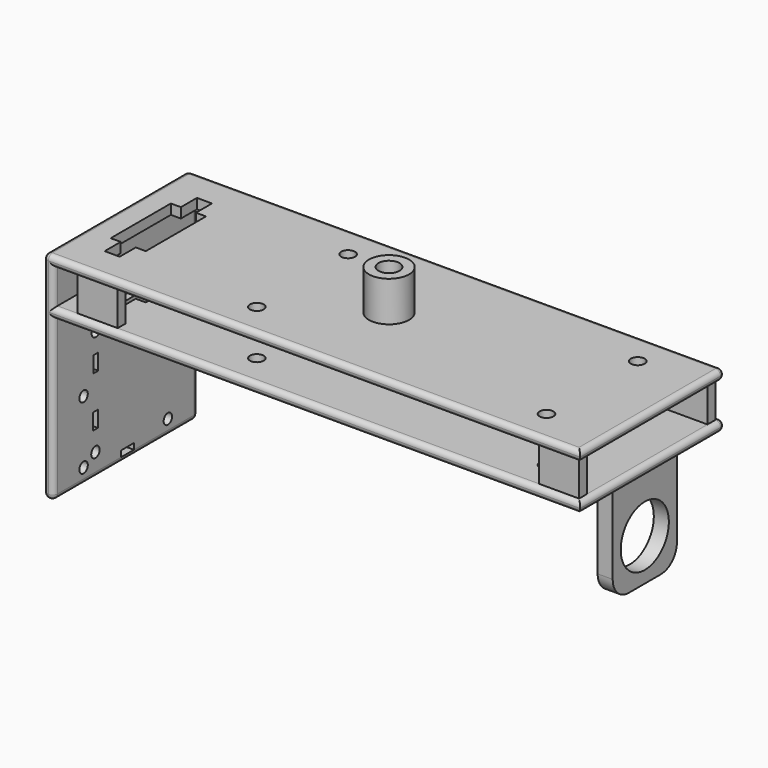
from build123d import *

# Parameters (mm, degrees)
F0_W      = 105
F0_H      = 2
F1_DEPTH  = 18
F2_R      = 4
F3_DEPTH  = 8
F4_R      = 2.1
F5_DEPTH  = 3.5
F6_R      = 1.05
F7_DEPTH  = 2
F8_R      = 1.375
F9_DEPTH  = 11
F10_W     = 3
F10_H     = 4
F11_DEPTH = 11
F12_R     = 0.99999
F13_W     = 3
F13_H     = 16
F14_DEPTH = 20
F15_R     = 4
F16_R     = 6
F17_DEPTH = 3
F18_W     = 1.2
F18_H     = 3.2
F18_W_2   = 3.2
F18_H_2   = 1.2
F18_R     = 1.05
F19_DEPTH = 2
F20_W     = 8
F20_H     = 2
F21_DEPTH = 11


# Not quite as in the source:
# - a fillet or chamfer is up to 0.001 mm smaller than in the source, because OpenCascade refuses the exact size


with BuildPart() as f1:
    # F0 (on Front) → F1 (new body, symmetric)
    with BuildSketch(Plane.XZ):
        Polygon((0, -2), (0, 0), (-2, 0), (-2, -43), (0, -43), (0, -11), (0, -9), align=None)
        with Locations((52.5, -1)):
            Rectangle(F0_W, F0_H)
        with Locations((52.5, -10)):
            Rectangle(F0_W, F0_H)
    extrude(amount=F1_DEPTH, both=True)

    # F2 (on face) → F3 (join)
    with BuildSketch(Plane.XY):
        with Locations((52.5, 0)):
            Circle(F2_R)
    extrude(amount=F3_DEPTH)

    # F4 (on face) → F5 (cut)
    with BuildSketch(Plane.XY.offset(8)):
        with Locations((52.5, 0)):
            Circle(F4_R)
    extrude(amount=-F5_DEPTH, mode=Mode.SUBTRACT)

    # F6 (on face) → F7 (cut, through all)
    with BuildSketch(Plane(origin=(-2, 0, 0), x_dir=(0, -1, 0), z_dir=(-1, 0, 0))):
        with Locations((-10.5, -40)):
            Circle(F6_R)
        with Locations((10.5, -40)):
            Circle(F6_R)
        with Locations((-10.5, -27.5)):
            Circle(F6_R)
        with Locations((10.5, -27.5)):
            Circle(F6_R)
    extrude(amount=-F7_DEPTH, mode=Mode.SUBTRACT)

    # F8 (on face) → F9 (cut, through all)
    with BuildSketch(Plane.XY):
        with Locations((35.25, 11.375)):
            Circle(F8_R)
        with Locations((35.25, -11.375)):
            Circle(F8_R)
        with Locations((93, 11.375)):
            Circle(F8_R)
        with Locations((93, -11.375)):
            Circle(F8_R)
    extrude(amount=-F9_DEPTH, mode=Mode.SUBTRACT)

    # F10 (on face) → F11 (cut, through all)
    with BuildSketch(Plane.XY):
        Polygon((5, 7.5), (3, 7.5), (3, -7.5), (5, -7.5), (8, -7.5), (10, -7.5), (10, 7.5), (8, 7.5), (6.5, 7.5), align=None)
        Polygon((5, 11.5), (5, 7.5), (6.5, 7.5), (8, 7.5), (8, 11.5), align=None)
        with Locations((6.5, -9.5)):
            Rectangle(F10_W, F10_H)
    extrude(amount=-F11_DEPTH, mode=Mode.SUBTRACT)

    # F12 (radius 1 in the source; OpenCascade refuses exactly that, so slightly less here)
    f12_edges = [f1.edges().sort_by_distance(p)[0] for p in [
        (-2, 0, 0),
        (51.5, -18, 0),
        (51.5, 18, 0),
        (105, 0, 0),
        (105, 0, -2),
        (105, 0, -9),
        (105, 0, -11),
        (52.5, -18, -9),
        (52.5, -18, -11),
        (52.5, -18, -2),
        (0, -18, -27),
        (-2, -18, -21.5),
        (0, 0, -43),
        (-1, -18, -43),
        (52.5, 18, -2),
        (52.5, 18, -9),
        (52.5, 18, -11),
        (105, 18, -1),
        (105, 18, -10),
        (0, 18, -27),
        (0, 18, -5.5),
        (-2, 18, -21.5),
        (-1, 18, -43),
        (-2, 0, -43),
        (0, -18, -5.5),
    ]]
    fillet(f12_edges, radius=F12_R)

    # F13 (on face) → F14 (join)
    with BuildSketch(Plane(origin=(0, 0, -11), x_dir=(1, 0, 0), z_dir=(0, 0, -1))):
        with Locations((102, 0)):
            Rectangle(F13_W, F13_H)
    extrude(amount=F14_DEPTH)

    # F15
    f15_edges = [f1.edges().sort_by_distance(p)[0] for p in [
        (102, -8, -31),
        (102, 8, -31),
    ]]
    fillet(f15_edges, radius=F15_R)

    # F16 (on face) → F17 (cut, through all)
    with BuildSketch(Plane.YZ.offset(103.5)):
        with Locations((0, -22.608)):
            Circle(F16_R)
    extrude(amount=-F17_DEPTH, mode=Mode.SUBTRACT)

    # F18 (on face) → F19 (cut, through all)
    with BuildSketch(Plane.YZ):
        with Locations((-7.45, -22.9)):
            Rectangle(F18_W, F18_H)
        with Locations((-7.55, -32.9)):
            Rectangle(F18_W, F18_H)
        with Locations((0.45, -41.4)):
            Rectangle(F18_W_2, F18_H_2)
        with Locations((0.55, -14.4)):
            Rectangle(F18_W_2, F18_H_2)
        with Locations((-7.45, -17.3)):
            Circle(F18_R)
        with Locations((-7.55, -38.5)):
            Circle(F18_R)
    extrude(amount=-F19_DEPTH, mode=Mode.SUBTRACT)

    # F20 (on face) → F21 (join, through all)
    with BuildSketch(Plane.XY):
        with Locations((17, 16)):
            Rectangle(F20_W, F20_H)
        with Locations((100, 16)):
            Rectangle(F20_W, F20_H)
        with Locations((100, -16)):
            Rectangle(F20_W, F20_H)
        with Locations((8, -16)):
            Rectangle(F20_W, F20_H)
    extrude(amount=-F21_DEPTH)


solid = f1.part
